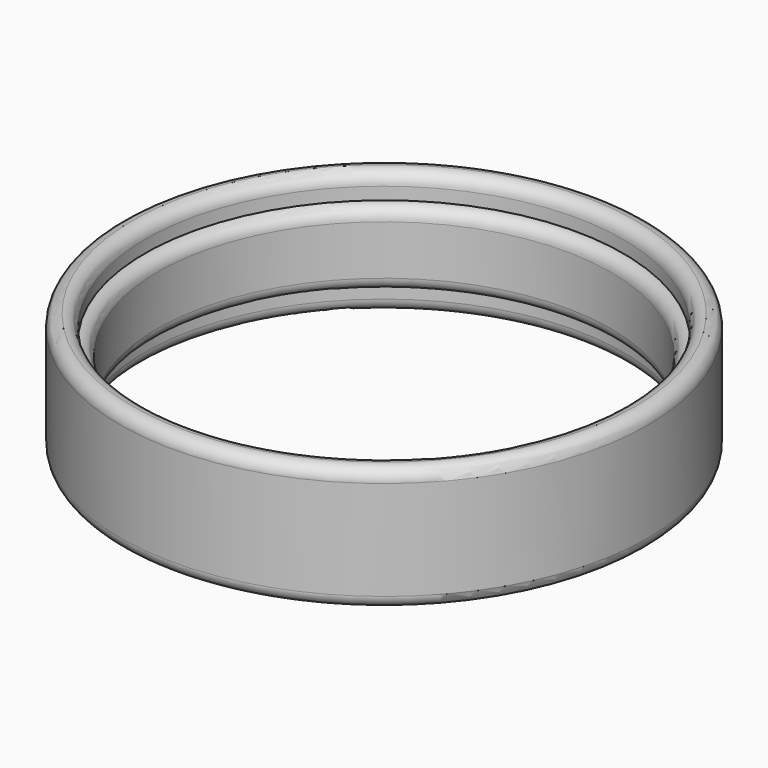
from build123d import *

# Parameters (mm, degrees)
F0_R     = 21.25
F0_R_2   = 19.25
F1_DEPTH = 10
F3_R     = 21.25
F3_R_2   = 18.25
F4_DEPTH = 6
F5_R     = 0.99999


# Not quite as in the source:
# - a fillet or chamfer is up to 0.001 mm smaller than in the source, because OpenCascade refuses the exact size


with BuildPart() as f1:
    # F0 (on Top) → F1 (new body)
    with BuildSketch(Plane.XY):
        Circle(F0_R)
        Circle(F0_R_2, mode=Mode.SUBTRACT)
    extrude(amount=F1_DEPTH)

    # F3 (on offset) → F4 (join)
    with BuildSketch(Plane.XY.offset(2)):
        Circle(F3_R)
        Circle(F3_R_2, mode=Mode.SUBTRACT)
    extrude(amount=F4_DEPTH)

    # F5 (radius 1 in the source; OpenCascade refuses exactly that, so slightly less here)
    f5_edges = [f1.edges().sort_by_distance(p)[0] for p in [
        (-18.25, 0, 2),
        (-18.25, 0, 8),
        (-19.25, 0, 10),
        (-21.25, 0, 10),
        (-21.25, 0, 0),
        (-19.25, 0, 0),
    ]]
    fillet(f5_edges, radius=F5_R)


solid = f1.part
